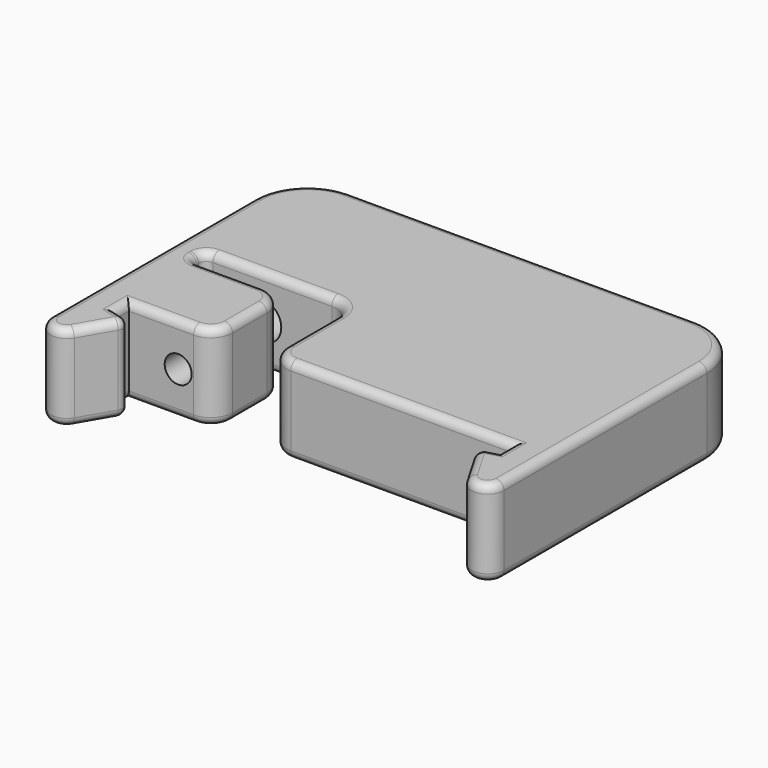
from build123d import *

# Parameters (mm, degrees)
F1_DEPTH    = 4
F2_R        = 1.25
F3_DEPTH    = 14.501
F4_R        = 1.75
F5_DEPTH    = 13.751
F7_R        = 3
F8_DEPTH    = 4.001
F9_T1_DEPTH = 33
F10_R       = 2
F11_R       = 0.75


# Not quite as in the source:
# - a fillet or chamfer that OpenCascade refuses, or shapes differently, is made with other operations: its cross-section is extruded or revolved along the edge and cut away or added


with BuildPart() as f1:
    # F0 (on Top) → F1 (new body, symmetric)
    with BuildSketch(Plane.XY):
        with BuildLine():
            Line((-17.75, -1.5), (-17.75, 0))
            Line((-17.75, 0), (-9.75, 0))
            Line((-9.75, 0), (-9.75, 8))
            Line((-9.75, 8), (-18.5, 8))
            Line((-18.5, 8), (-18.5, 9.75))
            Line((-18.5, 9.75), (-4.75, 9.75))
            Line((-4.75, 9.75), (-4.75, 0))
            Line((-4.75, 0), (17.75, 0))
            Line((17.75, 0), (17.75, -1.5))
            Line((17.75, -1.5), (16, -1.9689110868))
            Line((16, -1.9689110868), (18.2036332099, -5.7546079415))
            ThreePointArc((18.2036332099, -5.7546079415), (19.8908003421, -6.4481971871), (21, -5))
            Line((21, -5), (21, 23.5))
            Line((21, 23.5), (-21, 23.5))
            Line((-21, 23.5), (-21, -5))
            ThreePointArc((-21, -5), (-19.8908003421, -6.4481971871), (-18.2036332099, -5.7546079415))
            Line((-18.2036332099, -5.7546079415), (-16, -1.9689110868))
            Line((-16, -1.9689110868), (-17.75, -1.5))
        make_face()
    extrude(amount=F1_DEPTH, both=True)

    # F2 (on face) → F3 (cut, through all)
    with BuildSketch(Plane(origin=(0, 8, 0), x_dir=(-1, 0, 0), z_dir=(0, 1, 0))):
        with Locations((13.1794307381, 0)):
            Circle(F2_R)
    extrude(amount=-F3_DEPTH, mode=Mode.SUBTRACT)

    # F4 (on face) → F5 (cut, through all)
    with BuildSketch(Plane.XZ.offset(-9.75)):
        with Locations((-13.1794307381, 0)):
            Circle(F4_R)
    extrude(amount=-F5_DEPTH, mode=Mode.SUBTRACT)

    # F7 (on offset) → F8 (cut, through all)
    with BuildSketch(Plane(origin=(0, 19.5, 0), x_dir=(-1, 0, 0), z_dir=(0, 1, 0))):
        with Locations((13.1794307381, 0)):
            Circle(F7_R)
    extrude(amount=F8_DEPTH, mode=Mode.SUBTRACT)

    # F9: fillet of radius 5 on 2 edges, made by hand

    # F9_s2 → F9_t1 (cut)
    with BuildSketch(Plane.XY.offset(-16.5)):
        with BuildLine():
            ThreePointArc((-16, 23.5), (-19.5355339059, 22.0355339059), (-21, 18.5))
            Line((-21, 18.5), (-21, 23.5))
            Line((-21, 23.5), (-16, 23.5))
        make_face()
        with BuildLine():
            ThreePointArc((21, 18.5), (19.5355339059, 22.0355339059), (16, 23.5))
            Line((16, 23.5), (21, 23.5))
            Line((21, 23.5), (21, 18.5))
        make_face()
    extrude(amount=F9_T1_DEPTH, mode=Mode.SUBTRACT)

    # F10
    f10_edges = [f1.edges().sort_by_distance(p)[0] for p in [
        (-4.75, 0, 0),
        (-9.75, 0, 0),
        (-9.75, 8, 0),
        (-4.75, 9.75, 0),
    ]]
    fillet(f10_edges, radius=F10_R)

    # F11
    f11_edges = [f1.edges().sort_by_distance(p)[0] for p in [
        (-16, -1.968911, 0),
        (16, -1.968911, 0),
        (-18.5, 9.75, 0),
        (-18.5, 8, 0),
        (7.5, 0, 4),
        (-4.164214, 0.585786, 4),
        (17.75, -0.75, 4),
        (-4.75, 4.875, 4),
        (16.875, -1.734456, 4),
        (-5.335786, 9.164214, 4),
        (17.101817, -3.86176, 4),
        (-12.625, 9.75, 4),
        (19.8908, -6.448197, 4),
        (-18.5, 8.875, 4),
        (21, 6.75, 4),
        (-15.125, 8, 4),
        (19.535534, 22.035534, 4),
        (-10.335786, 7.414214, 4),
        (0, 23.5, 4),
        (-9.75, 4, 4),
        (-19.535534, 22.035534, 4),
        (-10.335786, 0.585786, 4),
        (-21, 6.75, 4),
        (-14.75, 0, 4),
        (-19.8908, -6.448197, 4),
        (-17.75, -0.75, 4),
        (-17.101817, -3.86176, 4),
        (-16.875, -1.734456, 4),
        (7.5, 0, -4),
        (-4.164214, 0.585786, -4),
        (17.75, -0.75, -4),
        (-4.75, 4.875, -4),
        (16.875, -1.734456, -4),
        (-5.335786, 9.164214, -4),
        (17.101817, -3.86176, -4),
        (-12.625, 9.75, -4),
        (19.8908, -6.448197, -4),
        (-18.5, 8.875, -4),
        (21, 6.75, -4),
        (-15.125, 8, -4),
        (19.535534, 22.035534, -4),
        (-10.335786, 7.414214, -4),
        (0, 23.5, -4),
        (-9.75, 4, -4),
        (-19.535534, 22.035534, -4),
        (-10.335786, 0.585786, -4),
        (-21, 6.75, -4),
        (-14.75, 0, -4),
        (-19.8908, -6.448197, -4),
        (-17.75, -0.75, -4),
        (-17.101817, -3.86176, -4),
        (-16.875, -1.734456, -4),
    ]]
    fillet(f11_edges, radius=F11_R)


solid = f1.part
